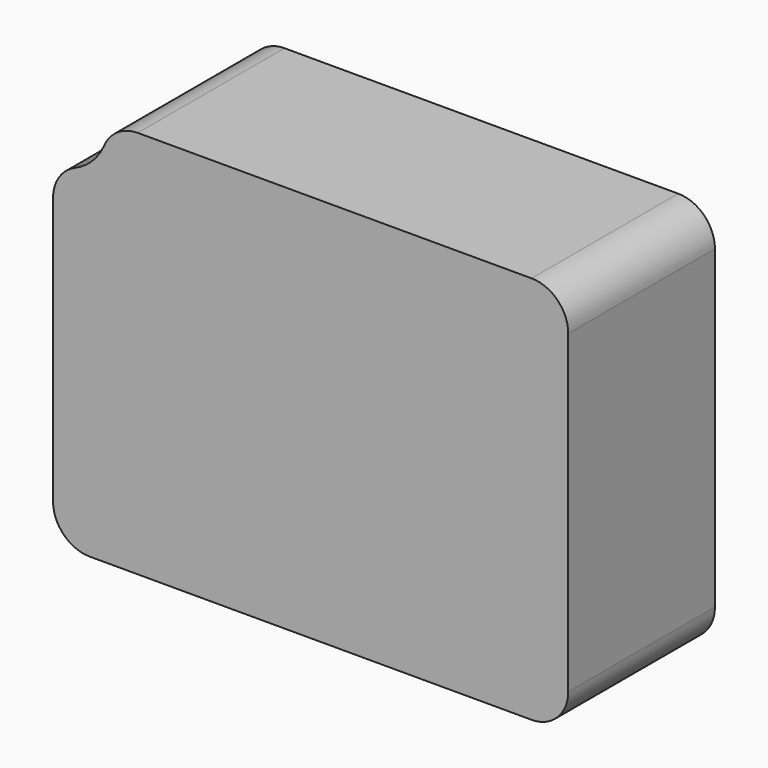
from build123d import *

# Parameters (mm, degrees)
F1_DEPTH = 25.4
F2_R     = 5.08


with BuildPart() as f1:
    # F0 (on Front) → F1 (new body)
    with BuildSketch(Plane.XZ):
        with BuildLine():
            Line((-35.6792770326, -26.9159432501), (35.6792770326, -26.9159432501))
            Line((35.6792770326, -26.9159432501), (35.6792770326, 26.9159432501))
            Line((35.6792770326, 26.9159432501), (-27.9675787613, 26.9159432501))
            ThreePointArc((-27.9675787613, 26.9159432501), (-30.2262828905, 21.462949108), (-35.6792770326, 19.2042449788))
            Line((-35.6792770326, 19.2042449788), (-35.6792770326, -26.9159432501))
        make_face()
    extrude(amount=F1_DEPTH)

    # F2
    f2_edges = [f1.edges().sort_by_distance(p)[0] for p in [
        (35.679277, -12.7, 26.915943),
        (-35.679277, -12.7, -26.915943),
        (35.679277, -12.7, -26.915943),
        (-35.679277, -12.7, 19.204245),
        (-27.967579, -12.7, 26.915943),
    ]]
    fillet(f2_edges, radius=F2_R)


solid = f1.part
